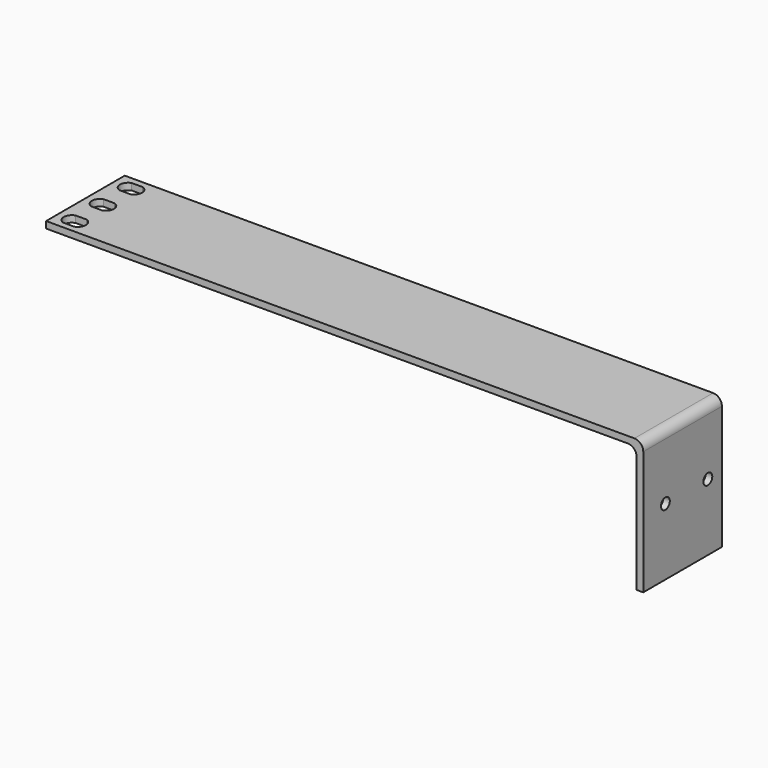
from build123d import *

# Parameters (mm, degrees)
F0_W     = 270
F0_H     = 44.45
F1_DEPTH = 3
F3_DEPTH = 3
F2_W     = 3
F2_H     = 44.45
F4_DEPTH = 60
F5_R     = 2.5
F6_DEPTH = 3
F7_R     = 4
F8_R     = 4


# Not quite as in the source:
# - a feature names something its author has since deleted; it is built from what else it names


with BuildPart() as f1:
    # F0 (on Top) → F1 (new body)
    with BuildSketch(Plane.XY):
        with Locations((68.0511838198, -14.3298729897)):
            Rectangle(F0_W, F0_H)
    extrude(amount=F1_DEPTH)

    # F2 (on face) → F3 (cut)
    with BuildSketch(Plane.XY.offset(3)):
        with BuildLine():
            Line((-56.5113161802, -26.720496912), (-59.0113161802, -26.720496912))
            Line((-59.0113161802, -26.720496912), (-61.5113161802, -26.720496912))
            ThreePointArc((-61.5113161802, -26.720496912), (-64.0113244271, -30.220496912), (-61.5113161802, -33.720496912))
            Line((-61.5113161802, -33.720496912), (-59.0113161802, -33.720496912))
            Line((-59.0113161802, -33.720496912), (-56.5113161802, -33.720496912))
            ThreePointArc((-56.5113161802, -33.720496912), (-54.0113161802, -30.220496912), (-56.5113161802, -26.720496912))
        make_face()
        with BuildLine():
            Line((-61.5113161802, -17.845496912), (-59.0113161802, -17.845496912))
            Line((-59.0113161802, -17.845496912), (-56.5113161802, -17.845496912))
            ThreePointArc((-56.5113161802, -17.845496912), (-54.0113161802, -14.345496912), (-56.5113161802, -10.845496912))
            Line((-56.5113161802, -10.845496912), (-59.0113161802, -10.845496912))
            Line((-59.0113161802, -10.845496912), (-61.5113161802, -10.845496912))
            ThreePointArc((-61.5113161802, -10.845496912), (-64.0113244271, -14.345496912), (-61.5113161802, -17.845496912))
        make_face()
        with BuildLine():
            Line((-61.5113161802, -1.970496912), (-59.0113161802, -1.970496912))
            Line((-59.0113161802, -1.970496912), (-56.5113161802, -1.970496912))
            ThreePointArc((-56.5113161802, -1.970496912), (-54.0113161802, 1.529503088), (-56.5113161802, 5.029503088))
            Line((-56.5113161802, 5.029503088), (-59.0113161802, 5.029503088))
            Line((-59.0113161802, 5.029503088), (-61.5113161802, 5.029503088))
            ThreePointArc((-61.5113161802, 5.029503088), (-64.0113244271, 1.529503088), (-61.5113161802, -1.970496912))
        make_face()
    extrude(amount=-F3_DEPTH, mode=Mode.SUBTRACT)

    # F2 (on face) → F4 (join)
    with BuildSketch(Plane.XY.offset(3)):
        with Locations((201.5511838198, -14.3298729897)):
            Rectangle(F2_W, F2_H)
    extrude(amount=-F4_DEPTH)

    # F5 (on face) → F6 (cut)
    with BuildSketch(Plane.YZ.offset(203.0511838198)):
        with Locations((-24.0548729897, -26.75)):
            Circle(F5_R)
        with Locations((-0.0548729897, -26.75)):
            Circle(F5_R)
    extrude(amount=-F6_DEPTH, mode=Mode.SUBTRACT)

    # F7
    f7_edges = [f1.edges().sort_by_distance(p)[0] for p in [
        (200.051184, -14.329873, 0),
    ]]
    fillet(f7_edges, radius=F7_R)

    # F8
    f8_edges = [f1.edges().sort_by_distance(p)[0] for p in [
        (203.051184, -14.329873, 3),
    ]]
    fillet(f8_edges, radius=F8_R)


solid = f1.part
